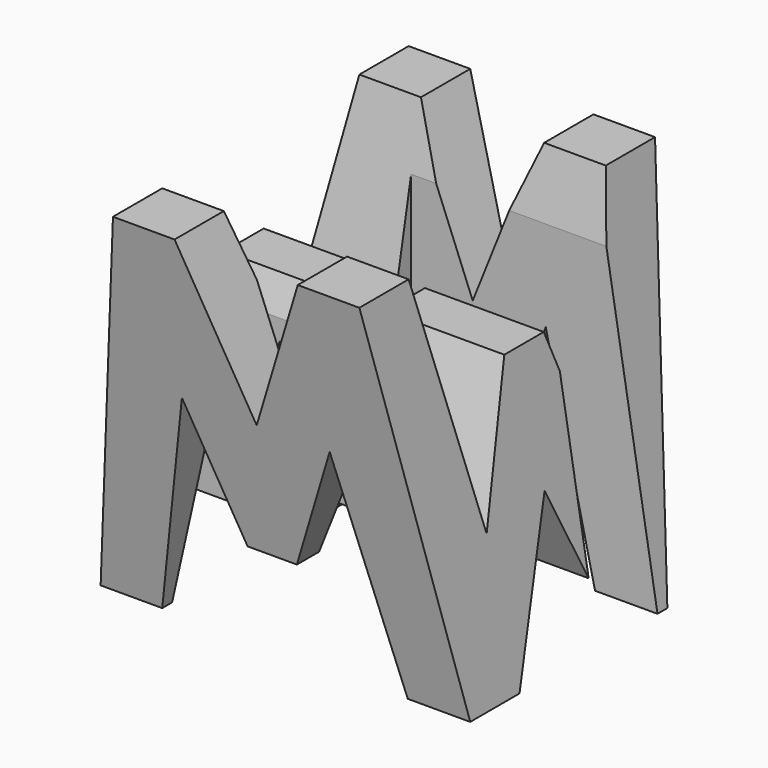
from build123d import *

# Parameters (mm, degrees)
F0_W      = 38.1
F0_H      = 38.1
F1_DEPTH  = 38.1
F6_DEPTH  = 38.1
F8_DEPTH  = 38.1
F9_W      = 25.4
F9_H      = 7.62
F10_DEPTH = 38.1


# Not quite as in the source:
# - a feature names something its author has since deleted; it is built from what else it names


with BuildPart() as f1:
    # F0 (on Front) → F1 (new body)
    with BuildSketch(Plane.XZ):
        with Locations((19.05, 19.05)):
            Rectangle(F0_W, F0_H)
    extrude(amount=F1_DEPTH)

    # F5 (on offset) → F6 (cut)
    with BuildSketch(Plane.YZ.offset(38.1)):
        Polygon((-11.43, 12.2219994664), (-6.35, 38.1), (-31.75, 38.1), (-26.67, 14.2379999161), (-21.59, 27.6940000847), (-16.51, 27.6940000847), align=None)
        Polygon((-31.75, 0), (-38.1, 38.1), (-38.1, 0), align=None)
        Polygon((-25.4, 0), (-19.05, 0), (-19.05, 14.9940000847), align=None)
        Polygon((-19.05, 0), (-12.7, 0), (-19.05, 14.9940000847), align=None)
        Polygon((-6.35, 0), (0, 0), (0, 38.1), align=None)
    extrude(amount=-F6_DEPTH, mode=Mode.SUBTRACT)

    # F7 (on offset) → F8 (cut)
    with BuildSketch(Plane.XZ.offset(38.1)):
        Polygon((0, 38.1), (0, 0), (6.35, 38.1), align=None)
        Polygon((25.4, 38.1), (12.7, 38.1), (19.05, 22.225), align=None)
        Polygon((31.75, 38.1), (38.1, 0), (38.1, 38.1), align=None)
        Polygon((11.340001598, 22.225), (6.35, 0), (31.660001598, 0), (26.580001598, 22.2758815411), (21.500001598, 9.525), (16.420001598, 9.525), align=None)
    extrude(amount=-F8_DEPTH, mode=Mode.SUBTRACT)

    # F9 (on offset) → F10 (cut)
    with BuildSketch(Plane.XY.offset(38.1)):
        with Locations((25.4, -11.43)):
            Rectangle(F9_W, F9_H)
        with Locations((12.7, -26.67)):
            Rectangle(F9_W, F9_H)
    extrude(amount=-F10_DEPTH, mode=Mode.SUBTRACT)


solid = f1.part
